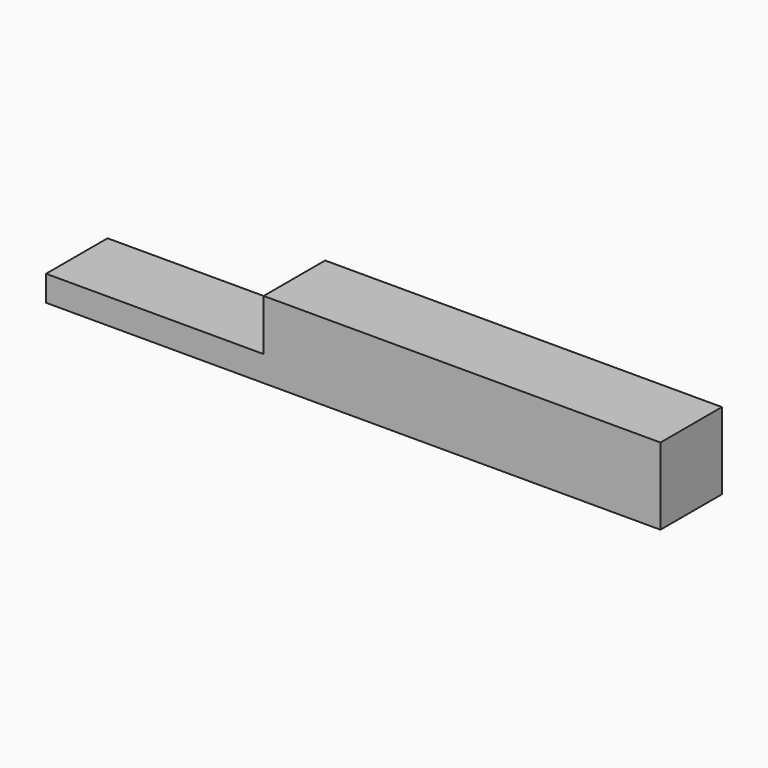
from build123d import *

# Parameters (mm, degrees)
F1_DEPTH = 12


# Not quite as in the source:
# - a feature names something its author has since deleted; it is built from what else it names


with BuildPart() as f1:
    # F0 (on Front) → F1 (new body)
    with BuildSketch(Plane.XZ):
        Polygon((55, -96), (21, -96), (21, -100), (117, -100), (117, -88), (55, -88), align=None)
    extrude(amount=-F1_DEPTH)


solid = f1.part
